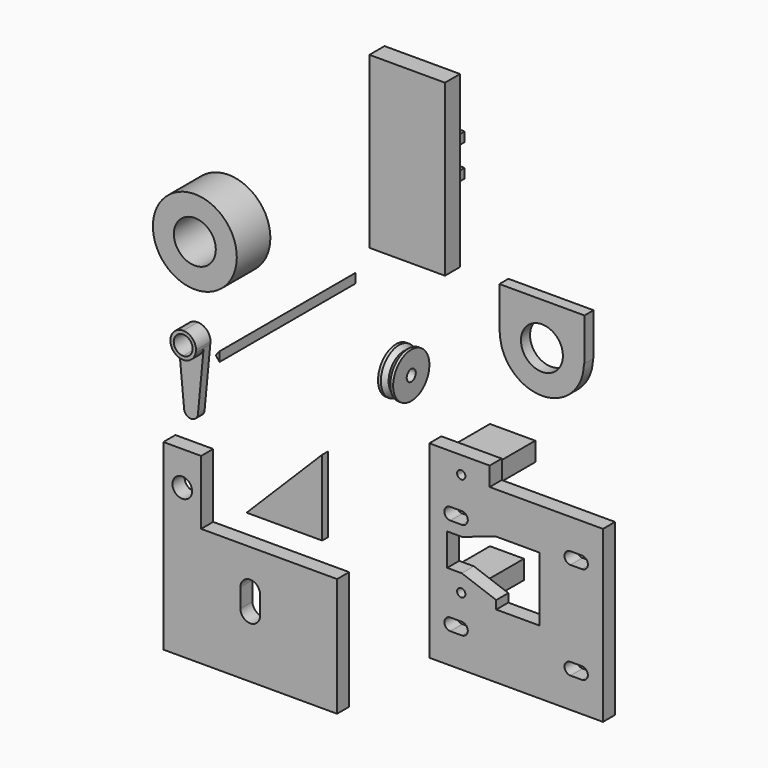
from build123d import *
from build123d import SkipClean  # not in build123d's __all__

# Parameters (mm, degrees)
F0_R      = 11.115
F0_R_2    = 5.555
F1_DEPTH  = 11.11
F4_DEPTH  = 4.8
F5_DEPTH  = 2.2
F0_W      = 9
F0_H      = 5
F0_R_3    = 1.1
F6_DEPTH  = 4
F7_DEPTH  = 3
F0_W_2    = 20
F0_H_2    = 45
F0_W_3    = 8
F0_H_3    = 2.5
F8_DEPTH  = 5
F9_DEPTH  = 14
F10_DEPTH = 45
F0_W_4    = 10
F0_H_4    = 17
F0_R_4    = 2.6
F11_DEPTH = 4
F12_DEPTH = 2
F13_DEPTH = 13


with BuildPart() as f1:
    # F0 (on Front) → F1 (new body)
    with BuildSketch(Plane.XZ):
        with Locations((-46.419493854, 28.7711881101)):
            Circle(F0_R)
        with Locations((-46.419493854, 28.7711881101)):
            Circle(F0_R_2, mode=Mode.SUBTRACT)
    extrude(amount=F1_DEPTH)


with BuildPart() as f3:
    # F2 (on Front) → F3 (revolve)
    with BuildSketch(Plane.XZ):
        Polygon((-2, 10.3620744314), (2, 10.3620744314), (2, 14.8620744314), (1.25, 14.8620744314), (0, 13.8620744314), (-1.25, 14.8620744314), (-2, 14.8620744314), align=None)
    revolve(axis=Axis((0, 0, 8.8620744314), (-1, 0, 0)))


with BuildPart() as f4:
    # F0 (on Front) → F4 (new body)
    with BuildSketch(Plane.XZ):
        with BuildLine():
            Line((-51.2152923013, -1.1903753393), (-51.1547232032, -0.5514690459))
            ThreePointArc((-51.1547232032, -0.5514690459), (-52.1505601471, 1.8526940102), (-54.5547232032, 2.8485309541))
            Line((-54.5547232032, 2.8485309541), (-54.5547232032, 1.9485309541))
            ThreePointArc((-54.5547232032, 1.9485309541), (-52.7869562502, 1.2162979071), (-52.0547232032, -0.5514690459))
            ThreePointArc((-52.0547232032, -0.5514690459), (-52.7869562502, -2.3192359988), (-54.5547232032, -3.0514690459))
            Line((-54.5547232032, -3.0514690459), (-54.5547232032, -3.9514690459))
            ThreePointArc((-54.5547232032, -3.9514690459), (-52.3881915738, -3.1718012193), (-51.2152923013, -1.1903753393))
        make_face()
        with BuildLine():
            Line((-54.5547232032, 1.9485309541), (-54.5547232032, 2.8485309541))
            ThreePointArc((-54.5547232032, 2.8485309541), (-56.9588862592, 1.8526940102), (-57.9547232032, -0.5514690459))
            Line((-57.9547232032, -0.5514690459), (-57.894154105, -1.1903753393))
            ThreePointArc((-57.894154105, -1.1903753393), (-56.7212548326, -3.1718012193), (-54.5547232032, -3.9514690459))
            Line((-54.5547232032, -3.9514690459), (-54.5547232032, -3.0514690459))
            ThreePointArc((-54.5547232032, -3.0514690459), (-57.0547232032, -0.5514690459), (-54.5547232032, 1.9485309541))
        make_face()
    extrude(amount=F4_DEPTH)

    # F0 (on Front) → F5 (join)
    with BuildSketch(Plane.XZ):
        with BuildLine():
            Line((-52.7047232032, -16.9014690459), (-51.2152923013, -1.1903753393))
            ThreePointArc((-51.2152923013, -1.1903753393), (-52.3881915738, -3.1718012193), (-54.5547232032, -3.9514690459))
            Line((-54.5547232032, -3.9514690459), (-54.5547232032, -15.0514690459))
            ThreePointArc((-54.5547232032, -15.0514690459), (-53.246575658, -15.5933215007), (-52.7047232032, -16.9014690459))
        make_face()
        with BuildLine():
            Line((-54.5547232032, -15.0514690459), (-54.5547232032, -3.9514690459))
            ThreePointArc((-54.5547232032, -3.9514690459), (-56.7212548326, -3.1718012193), (-57.894154105, -1.1903753393))
            Line((-57.894154105, -1.1903753393), (-56.4047232032, -16.9014690459))
            ThreePointArc((-56.4047232032, -16.9014690459), (-55.8628707484, -15.5933215007), (-54.5547232032, -15.0514690459))
        make_face()
        with BuildLine():
            ThreePointArc((-54.5547232032, -18.7514690459), (-53.246575658, -18.2096165911), (-52.7047232032, -16.9014690459))
            ThreePointArc((-52.7047232032, -16.9014690459), (-53.246575658, -15.5933215007), (-54.5547232032, -15.0514690459))
            Line((-54.5547232032, -15.0514690459), (-54.5547232032, -18.7514690459))
        make_face()
        with BuildLine():
            Line((-54.5547232032, -18.7514690459), (-54.5547232032, -15.0514690459))
            ThreePointArc((-54.5547232032, -15.0514690459), (-55.8628707484, -15.5933215007), (-56.4047232032, -16.9014690459))
            ThreePointArc((-56.4047232032, -16.9014690459), (-55.8628707484, -18.2096165911), (-54.5547232032, -18.7514690459))
        make_face()
    extrude(amount=F5_DEPTH)


with BuildPart() as f5:
    # F0 (on Front) → F5, piece 2 (new body)
    with BuildSketch(Plane.XZ):
        Polygon((55.9720356852, -7.7514690459), (25.9720356852, -7.7514690459), (24.442558834, -7.7514690459), (24.442558834, -9.3514690459), (12.442558834, -9.3514690459), (12.442558834, -7.7514690459), (9.9720356852, -7.7514690459), (9.9720356852, -52.7514690459), (55.9720356852, -52.7514690459), align=None)
        with BuildLine():
            ThreePointArc((15.5720356852, -44.7514690459), (13.9720356852, -43.1514690459), (15.5720356852, -41.5514690459))
            Line((15.5720356852, -41.5514690459), (18.5720356852, -41.5514690459))
            ThreePointArc((18.5720356852, -41.5514690459), (19.7034065351, -42.020098196), (20.1720356852, -43.1514690459))
            ThreePointArc((20.1720356852, -43.1514690459), (19.7034065351, -44.2828398958), (18.5720356852, -44.7514690459))
            Line((18.5720356852, -44.7514690459), (15.5720356852, -44.7514690459))
        make_face(mode=Mode.SUBTRACT)
        with Locations((16.9430356852, -35.3514690459)):
            Rectangle(F0_W, F0_H, mode=Mode.SUBTRACT)
        with BuildLine():
            ThreePointArc((47.3720356852, -44.7514690459), (45.7720356852, -43.1514690459), (47.3720356852, -41.5514690459))
            Line((47.3720356852, -41.5514690459), (50.3720356852, -41.5514690459))
            ThreePointArc((50.3720356852, -41.5514690459), (51.5034065351, -42.020098196), (51.9720356852, -43.1514690459))
            ThreePointArc((51.9720356852, -43.1514690459), (51.5034065351, -44.2828398958), (50.3720356852, -44.7514690459))
            Line((50.3720356852, -44.7514690459), (47.3720356852, -44.7514690459))
        make_face(mode=Mode.SUBTRACT)
        with BuildLine():
            ThreePointArc((15.5720356852, -18.9514690459), (13.9720356852, -17.3514690459), (15.5720356852, -15.7514690459))
            Line((15.5720356852, -15.7514690459), (18.5720356852, -15.7514690459))
            ThreePointArc((18.5720356852, -15.7514690459), (19.7034065351, -16.220098196), (20.1720356852, -17.3514690459))
            ThreePointArc((20.1720356852, -17.3514690459), (19.7034065351, -18.4828398958), (18.5720356852, -18.9514690459))
            Line((18.5720356852, -18.9514690459), (15.5720356852, -18.9514690459))
        make_face(mode=Mode.SUBTRACT)
        Polygon((18.5947939754, -21.7514690459), (27.7076829225, -18.7514690459), (39.2076829225, -18.7514690459), (39.2076829225, -35.7514690459), (27.7076829225, -35.7514690459), (27.7076829225, -33.5322953761), (18.5947939754, -30.2514690459), (14.7076829225, -30.2514690459), (14.7076829225, -21.7514690459), align=None, mode=Mode.SUBTRACT)
        with BuildLine():
            ThreePointArc((47.3720356852, -18.9514690459), (45.7720356852, -17.3514690459), (47.3720356852, -15.7514690459))
            Line((47.3720356852, -15.7514690459), (50.3720356852, -15.7514690459))
            ThreePointArc((50.3720356852, -15.7514690459), (51.5034065351, -16.220098196), (51.9720356852, -17.3514690459))
            ThreePointArc((51.9720356852, -17.3514690459), (51.5034065351, -18.4828398958), (50.3720356852, -18.9514690459))
            Line((50.3720356852, -18.9514690459), (47.3720356852, -18.9514690459))
        make_face(mode=Mode.SUBTRACT)
    extrude(amount=F5_DEPTH)

    # F0 (on Front) → F6 (join)
    with BuildSketch(Plane.XZ):
        Polygon((24.442558834, -7.7514690459), (25.9720356852, -7.7514690459), (25.9720356852, -2.7514690459), (9.9720356852, -2.7514690459), (9.9720356852, -7.7514690459), (12.442558834, -7.7514690459), (12.442558834, -4.3514690459), (24.442558834, -4.3514690459), align=None)
        with BuildLine():
            Line((19.4672539106, -7.7514690459), (24.442558834, -7.7514690459))
            Line((24.442558834, -7.7514690459), (24.442558834, -4.3514690459))
            Line((24.442558834, -4.3514690459), (12.442558834, -4.3514690459))
            Line((12.442558834, -4.3514690459), (12.442558834, -7.7514690459))
            Line((12.442558834, -7.7514690459), (17.4178637574, -7.7514690459))
            ThreePointArc((17.4178637574, -7.7514690459), (18.2390454244, -6.2704591976), (19.542558834, -7.3514690459))
            ThreePointArc((19.542558834, -7.3514690459), (19.5235686823, -7.5549824554), (19.4672539106, -7.7514690459))
        make_face()
        with BuildLine():
            Line((24.442558834, -9.3514690459), (24.442558834, -7.7514690459))
            Line((24.442558834, -7.7514690459), (19.4672539106, -7.7514690459))
            ThreePointArc((19.4672539106, -7.7514690459), (18.442558834, -8.4514690459), (17.4178637574, -7.7514690459))
            Line((17.4178637574, -7.7514690459), (12.442558834, -7.7514690459))
            Line((12.442558834, -7.7514690459), (12.442558834, -9.3514690459))
            Line((12.442558834, -9.3514690459), (24.442558834, -9.3514690459))
        make_face()
        Polygon((55.9720356852, -7.7514690459), (25.9720356852, -7.7514690459), (24.442558834, -7.7514690459), (24.442558834, -9.3514690459), (12.442558834, -9.3514690459), (12.442558834, -7.7514690459), (9.9720356852, -7.7514690459), (9.9720356852, -52.7514690459), (55.9720356852, -52.7514690459), align=None)
        with BuildLine():
            ThreePointArc((15.5720356852, -44.7514690459), (13.9720356852, -43.1514690459), (15.5720356852, -41.5514690459))
            Line((15.5720356852, -41.5514690459), (18.5720356852, -41.5514690459))
            ThreePointArc((18.5720356852, -41.5514690459), (19.7034065351, -42.020098196), (20.1720356852, -43.1514690459))
            ThreePointArc((20.1720356852, -43.1514690459), (19.7034065351, -44.2828398958), (18.5720356852, -44.7514690459))
            Line((18.5720356852, -44.7514690459), (15.5720356852, -44.7514690459))
        make_face(mode=Mode.SUBTRACT)
        with Locations((16.9430356852, -35.3514690459)):
            Rectangle(F0_W, F0_H, mode=Mode.SUBTRACT)
        with BuildLine():
            ThreePointArc((47.3720356852, -44.7514690459), (45.7720356852, -43.1514690459), (47.3720356852, -41.5514690459))
            Line((47.3720356852, -41.5514690459), (50.3720356852, -41.5514690459))
            ThreePointArc((50.3720356852, -41.5514690459), (51.5034065351, -42.020098196), (51.9720356852, -43.1514690459))
            ThreePointArc((51.9720356852, -43.1514690459), (51.5034065351, -44.2828398958), (50.3720356852, -44.7514690459))
            Line((50.3720356852, -44.7514690459), (47.3720356852, -44.7514690459))
        make_face(mode=Mode.SUBTRACT)
        with BuildLine():
            ThreePointArc((15.5720356852, -18.9514690459), (13.9720356852, -17.3514690459), (15.5720356852, -15.7514690459))
            Line((15.5720356852, -15.7514690459), (18.5720356852, -15.7514690459))
            ThreePointArc((18.5720356852, -15.7514690459), (19.7034065351, -16.220098196), (20.1720356852, -17.3514690459))
            ThreePointArc((20.1720356852, -17.3514690459), (19.7034065351, -18.4828398958), (18.5720356852, -18.9514690459))
            Line((18.5720356852, -18.9514690459), (15.5720356852, -18.9514690459))
        make_face(mode=Mode.SUBTRACT)
        Polygon((18.5947939754, -21.7514690459), (27.7076829225, -18.7514690459), (39.2076829225, -18.7514690459), (39.2076829225, -35.7514690459), (27.7076829225, -35.7514690459), (27.7076829225, -33.5322953761), (18.5947939754, -30.2514690459), (14.7076829225, -30.2514690459), (14.7076829225, -21.7514690459), align=None, mode=Mode.SUBTRACT)
        with BuildLine():
            ThreePointArc((47.3720356852, -18.9514690459), (45.7720356852, -17.3514690459), (47.3720356852, -15.7514690459))
            Line((47.3720356852, -15.7514690459), (50.3720356852, -15.7514690459))
            ThreePointArc((50.3720356852, -15.7514690459), (51.5034065351, -16.220098196), (51.9720356852, -17.3514690459))
            ThreePointArc((51.9720356852, -17.3514690459), (51.5034065351, -18.4828398958), (50.3720356852, -18.9514690459))
            Line((50.3720356852, -18.9514690459), (47.3720356852, -18.9514690459))
        make_face(mode=Mode.SUBTRACT)
        with Locations((16.9430356852, -35.3514690459)):
            Rectangle(F0_W, F0_H)
        with Locations((18.4430356852, -34.8514690459)):
            Circle(F0_R_3, mode=Mode.SUBTRACT)
    extrude(amount=F6_DEPTH)

    # F0 (on Front) → F13 (join)
    with BuildSketch(Plane.XZ):
        with BuildLine():
            Line((19.4672539106, -7.7514690459), (24.442558834, -7.7514690459))
            Line((24.442558834, -7.7514690459), (24.442558834, -4.3514690459))
            Line((24.442558834, -4.3514690459), (12.442558834, -4.3514690459))
            Line((12.442558834, -4.3514690459), (12.442558834, -7.7514690459))
            Line((12.442558834, -7.7514690459), (17.4178637574, -7.7514690459))
            ThreePointArc((17.4178637574, -7.7514690459), (18.2390454244, -6.2704591976), (19.542558834, -7.3514690459))
            ThreePointArc((19.542558834, -7.3514690459), (19.5235686823, -7.5549824554), (19.4672539106, -7.7514690459))
        make_face()
        with BuildLine():
            Line((24.442558834, -9.3514690459), (24.442558834, -7.7514690459))
            Line((24.442558834, -7.7514690459), (19.4672539106, -7.7514690459))
            ThreePointArc((19.4672539106, -7.7514690459), (18.442558834, -8.4514690459), (17.4178637574, -7.7514690459))
            Line((17.4178637574, -7.7514690459), (12.442558834, -7.7514690459))
            Line((12.442558834, -7.7514690459), (12.442558834, -9.3514690459))
            Line((12.442558834, -9.3514690459), (24.442558834, -9.3514690459))
        make_face()
        with Locations((16.9430356852, -35.3514690459)):
            Rectangle(F0_W, F0_H)
        with Locations((18.4430356852, -34.8514690459)):
            Circle(F0_R_3, mode=Mode.SUBTRACT)
    with SkipClean():  # cleaning this boolean's faces spoils the solid; the shape is the same uncleaned
        extrude(amount=-F13_DEPTH)


with BuildPart() as f5b:
    # F0 (on Front) → F5, piece 3 (new body)
    with BuildSketch(Plane.XZ):
        Polygon((-50.4410991073, -42.3525746226), (-60.4410991073, -42.3525746226), (-60.4410991073, -73.7525746226), (-14.4410991073, -73.7525746226), (-14.4410991073, -42.3525746226), align=None)
        with BuildLine():
            ThreePointArc((-34.8410991073, -57.5525746226), (-37.4410991073, -60.1525746226), (-40.0410991073, -57.5525746226))
            Line((-40.0410991073, -57.5525746226), (-40.0410991073, -52.5525746226))
            ThreePointArc((-40.0410991073, -52.5525746226), (-37.4410991073, -49.9525746226), (-34.8410991073, -52.5525746226))
            Line((-34.8410991073, -52.5525746226), (-34.8410991073, -57.5525746226))
        make_face(mode=Mode.SUBTRACT)
    extrude(amount=F5_DEPTH)

    # F0 (on Front) → F11 (join)
    with BuildSketch(Plane.XZ):
        Polygon((-50.4410991073, -42.3525746226), (-60.4410991073, -42.3525746226), (-60.4410991073, -73.7525746226), (-14.4410991073, -73.7525746226), (-14.4410991073, -42.3525746226), align=None)
        with BuildLine():
            ThreePointArc((-34.8410991073, -57.5525746226), (-37.4410991073, -60.1525746226), (-40.0410991073, -57.5525746226))
            Line((-40.0410991073, -57.5525746226), (-40.0410991073, -52.5525746226))
            ThreePointArc((-40.0410991073, -52.5525746226), (-37.4410991073, -49.9525746226), (-34.8410991073, -52.5525746226))
            Line((-34.8410991073, -52.5525746226), (-34.8410991073, -57.5525746226))
        make_face(mode=Mode.SUBTRACT)
        with Locations((-55.4410991073, -33.8525746226)):
            Rectangle(F0_W_4, F0_H_4)
        with Locations((-55.4410991073, -34.3525746226)):
            Circle(F0_R_4, mode=Mode.SUBTRACT)
    extrude(amount=F11_DEPTH)


with BuildPart() as f7:
    # F0 (on Front) → F7 (new body)
    with BuildSketch(Plane.XZ):
        with BuildLine():
            ThreePointArc((27.889240185, 28.4745767713), (39.004240185, 17.3595767713), (50.119240185, 28.4745767713))
            Line((50.119240185, 28.4745767713), (44.559240185, 28.4745767713))
            ThreePointArc((44.559240185, 28.4745767713), (39.004240185, 22.9195767713), (33.449240185, 28.4745767713))
            Line((33.449240185, 28.4745767713), (27.889240185, 28.4745767713))
        make_face()
        with BuildLine():
            ThreePointArc((27.889240185, 28.4745767713), (39.004240185, 39.5895767713), (50.119240185, 28.4745767713))
            Line((50.119240185, 28.4745767713), (50.2754300833, 28.4745767713))
            Line((50.2754300833, 28.4745767713), (50.2754300833, 39.7457666695))
            Line((50.2754300833, 39.7457666695), (27.7330502868, 39.7457666695))
            Line((27.7330502868, 39.7457666695), (27.7330502868, 28.4745767713))
            Line((27.7330502868, 28.4745767713), (27.889240185, 28.4745767713))
        make_face()
        with BuildLine():
            Line((44.559240185, 28.4745767713), (50.119240185, 28.4745767713))
            ThreePointArc((50.119240185, 28.4745767713), (39.004240185, 39.5895767713), (27.889240185, 28.4745767713))
            Line((27.889240185, 28.4745767713), (33.449240185, 28.4745767713))
            ThreePointArc((33.449240185, 28.4745767713), (39.004240185, 34.0295767713), (44.559240185, 28.4745767713))
        make_face()
    extrude(amount=F7_DEPTH)


with BuildPart() as f8:
    # F0 (on Front) → F8 (new body)
    with BuildSketch(Plane.XZ):
        with Locations((0.9291770309, 57.4878966808)):
            Rectangle(F0_W_2, F0_H_2)
        with Locations((0.9291770309, 51.2378966808)):
            Rectangle(F0_W_3, F0_H_3, mode=Mode.SUBTRACT)
        with Locations((0.9291770309, 59.7378966808)):
            Rectangle(F0_W_3, F0_H_3, mode=Mode.SUBTRACT)
    extrude(amount=-F8_DEPTH)

    # F0 (on Front) → F9 (join)
    with BuildSketch(Plane.XZ):
        with Locations((0.9291770309, 59.7378966808)):
            Rectangle(F0_W_3, F0_H_3)
        with Locations((0.9291770309, 51.2378966808)):
            Rectangle(F0_W_3, F0_H_3)
    extrude(amount=-F9_DEPTH)


with BuildPart() as f10:
    # F0 (on Front) → F10 (new body)
    with BuildSketch(Plane.XZ):
        Polygon((-12.762309216, 25.4634767771), (-12.762309216, 27.9634767771), (-13.762309216, 26.7134767771), align=None)
    extrude(amount=F10_DEPTH)


with BuildPart() as f12:
    # F0 (on Front) → F12 (new body)
    with BuildSketch(Plane.XZ):
        Polygon((-40, -35.9951816499), (-20, -35.9951816499), (-20, -15.9951816499), align=None)
    extrude(amount=F12_DEPTH)


solid = Compound([f1.part, f3.part, f4.part, f5.part, f5b.part, f7.part, f8.part, f10.part, f12.part])
